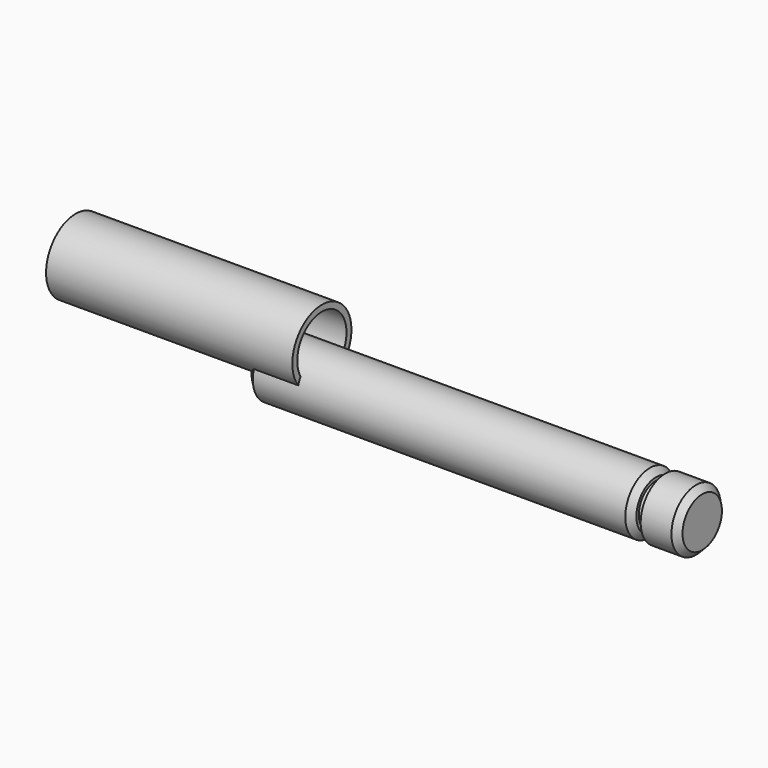
from build123d import *

# Parameters (mm, degrees)
F2_SIZE = 1


with BuildPart() as f1:
    # F0 (on Front) → F1 (revolve)
    with BuildSketch(Plane.XZ):
        Polygon((-83.1480100751, 5), (-83.1480100751, 0), (-74.9320751429, 0), (-13.1480100751, 0), (-13.1480100751, 5), (-19.1480100751, 5), (-19.1480100751, 3.5), (-20.6480100751, 3.5), (-20.6480100751, 5), (-74.9320751429, 5), align=None)
    revolve(axis=Axis((-48.1480100751, 0, 0), (1, 0, 0)))

    # F2
    f2_edges = [f1.edges().sort_by_distance(p)[0] for p in [
        (-13.14801, 0, -5),
        (-20.64801, 0, -5),
        (-83.14801, 0, -5),
    ]]
    chamfer(f2_edges, length=F2_SIZE)


with BuildPart() as f3:
    # F0 (on Front) → F3 (revolve)
    with BuildSketch(Plane.XZ):
        Polygon((-74.9320751429, 0), (-83.1480100751, 0), (-112.7974465489, 0), (-112.7974465489, -1), (-74.9320751429, -1), align=None)
        Polygon((-112.7974465489, -1), (-112.7974465489, 0), (-112.7974465489, 5), (-114.9320751429, 5), (-114.9320751429, 0), (-114.9320751429, -1), align=None)
    revolve(axis=Axis((-94.9320751429, 0, 5), (-1, 0, 0)))


solid = Compound([f1.part, f3.part])
